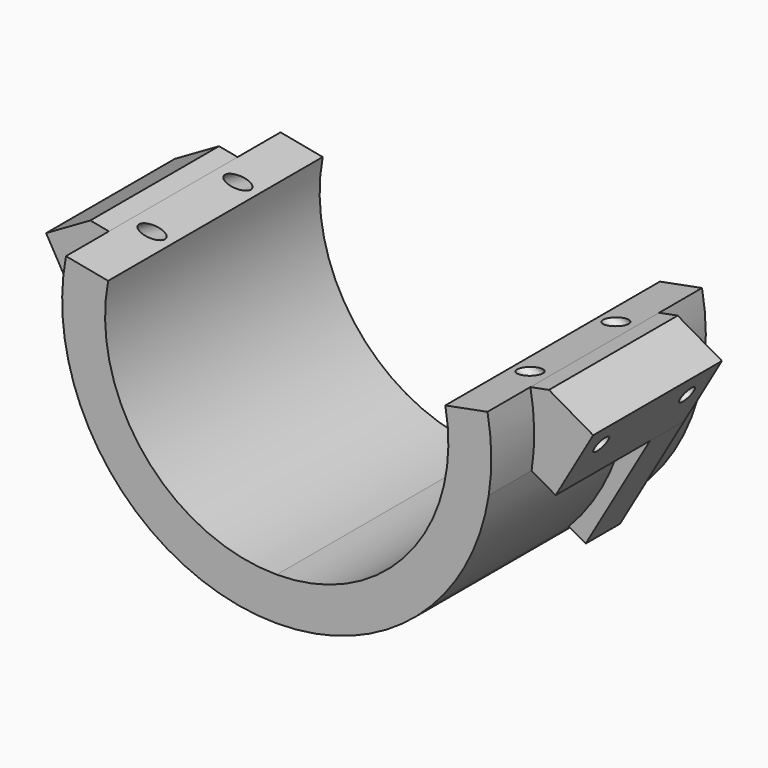
from build123d import *

# Parameters (mm, degrees)
F1_DEPTH = 20
F2_DEPTH = 5
F3_DEPTH = 4
F4_DEPTH = 15
F5_R     = 0.8
F6_DEPTH = 8.5841977808


# Not quite as in the source:
# - a feature names something its author has since deleted; it is built from what else it names


with BuildPart() as f1:
    # F0 (on Front) → F1 (new body)
    with BuildSketch(Plane.XZ):
        with BuildLine():
            ThreePointArc((15.7162336455, 3), (12.3288280059, -10.1980390272), (0, -16))
            Line((0, -16), (0, -20))
            ThreePointArc((0, -20), (7.8433854689, -18.397861408), (14.4301518825, -13.8481304387))
            ThreePointArc((14.4301518825, -13.8481304387), (17.9256749339, -8.8696210836), (19.762883185, -3.0705778311))
            ThreePointArc((19.762883185, -3.0705778311), (19.9970282657, 0.3447615687), (19.6452920569, 3.75))
            Line((19.6452920569, 3.75), (15.7162336455, 3))
        make_face()
    extrude(amount=F1_DEPTH)

    # F1_face (on face) → F2 (join)
    with BuildSketch(Plane(origin=(12.1989359317, 0, -10.0905961752), x_dir=(1, 0, 0), z_dir=(0, 1, 0))):
        with BuildLine():
            Line((3.5172977138, -13.0905961752), (7.4463561252, -13.8405961752))
            ThreePointArc((7.4463561252, -13.8405961752), (3.2120990757, 2.6569526088), (-12.1989359317, 9.9094038248))
            Line((-12.1989359317, 9.9094038248), (-12.1989359317, 5.9094038248))
            ThreePointArc((-12.1989359317, 5.9094038248), (0.1298920742, 0.107442852), (3.5172977138, -13.0905961752))
        make_face()
    extrude(amount=F2_DEPTH)

    # F0 (on Front) → F3 (join)
    with BuildSketch(Plane.XZ):
        with BuildLine():
            ThreePointArc((15.7162336455, 3), (12.3288280059, -10.1980390272), (0, -16))
            Line((0, -16), (0, -20))
            ThreePointArc((0, -20), (7.8433854689, -18.397861408), (14.4301518825, -13.8481304387))
            ThreePointArc((14.4301518825, -13.8481304387), (17.9256749339, -8.8696210836), (19.762883185, -3.0705778311))
            ThreePointArc((19.762883185, -3.0705778311), (19.9970282657, 0.3447615687), (19.6452920569, 3.75))
            Line((19.6452920569, 3.75), (15.7162336455, 3))
        make_face()
        with BuildLine():
            Line((21.3768143102, 4.080522368), (19.6452920569, 3.75))
            ThreePointArc((19.6452920569, 3.75), (19.9970282657, 0.3447615687), (19.762883185, -3.0705778311))
            Line((19.762883185, -3.0705778311), (22, -4.3621778265))
            Line((22, -4.3621778265), (25.5, 1.7))
            Line((25.5, 1.7), (21.3768143102, 4.080522368))
        make_face()
        with BuildLine():
            ThreePointArc((19.762883185, -3.0705778311), (17.9256749339, -8.8696210836), (14.4301518825, -13.8481304387))
            Line((14.4301518825, -13.8481304387), (16, -14.7544826719))
            Line((16, -14.7544826719), (22, -4.3621778265))
            Line((22, -4.3621778265), (19.762883185, -3.0705778311))
        make_face()
    extrude(amount=F3_DEPTH)

    # F0 (on Front) → F4 (join)
    with BuildSketch(Plane.XZ):
        with BuildLine():
            Line((21.3768143102, 4.080522368), (19.6452920569, 3.75))
            ThreePointArc((19.6452920569, 3.75), (19.9970282657, 0.3447615687), (19.762883185, -3.0705778311))
            Line((19.762883185, -3.0705778311), (22, -4.3621778265))
            Line((22, -4.3621778265), (25.5, 1.7))
            Line((25.5, 1.7), (21.3768143102, 4.080522368))
        make_face()
    extrude(amount=F4_DEPTH)

    # F5 (on face) → F6 (cut, through all)
    with BuildSketch(Plane(origin=(18.3888784068, 0, -10.6168238983), x_dir=(0, 1, 0), z_dir=(0.8660254038, 0, -0.5))):
        with Locations((-12.5, 11.7222431864)):
            Circle(F5_R)
        with Locations((-2.5, 11.7222431864)):
            Circle(F5_R)
    extrude(amount=-F6_DEPTH, mode=Mode.SUBTRACT)

    # F7: F1 across plane


with BuildPart() as f1_1:
    add(f1.part)
    add(f1.part.mirror(Plane.YZ))


solid = f1_1.part
